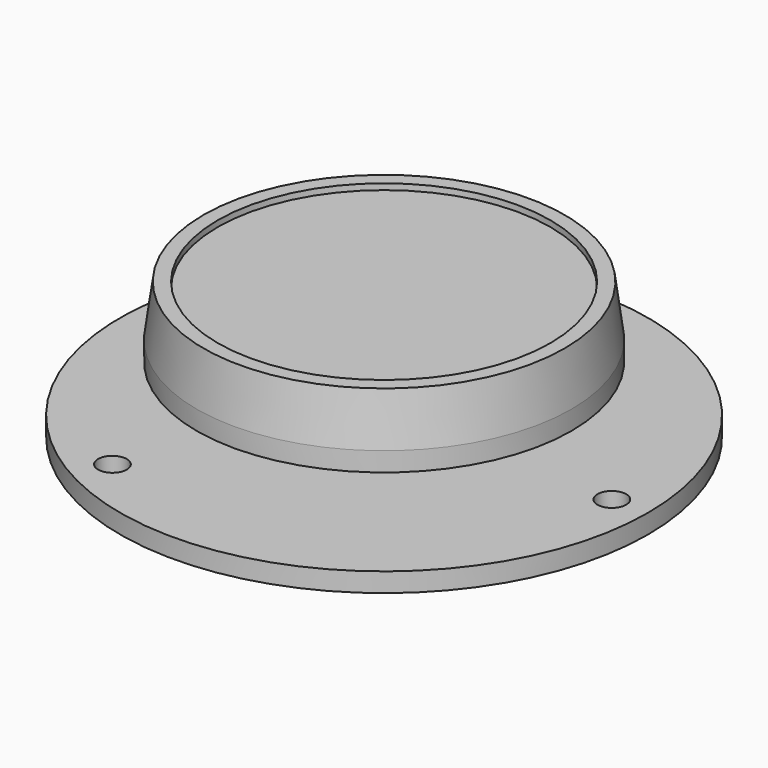
from build123d import *

# Parameters (mm, degrees)
F0_R            = 87.5
F0_R_2          = 10
F0_R_3          = 4.7625
F1_DEPTH        = 6.35
F2_DEPTH        = 6.35
F2_COPIES_COUNT = 3


# Not quite as in the source:
# - a length typed as a fraction of an inch, garbled in the dataset ("3 / 203.2 mm" for 3/8 in), is restored
# - a pattern or mirror of a feature is missing from the dataset's text; its kind, count and spacing are read off the source's solid
# - a feature names something its author has since deleted; it is built from what else it names


with BuildPart() as f1:
    # F0 (on Top) → F1 (new body)
    with BuildSketch(Plane.XY):
        Circle(F0_R)
        Circle(F0_R_2, mode=Mode.SUBTRACT)
        with Locations((75.5, 0)):
            Circle(F0_R_3, mode=Mode.SUBTRACT)
        with Locations((75.5, 0)):
            Circle(F0_R_3)
    extrude(amount=-F1_DEPTH)

    # F0 (on Top) → F2 (cut, through all)
    with BuildSketch(Plane.XY):
        with Locations((75.5, 0)):
            Circle(F0_R_3)
    f2 = extrude(amount=-F2_DEPTH, mode=Mode.SUBTRACT)

    # F2_copies: F2 ×3 about axis
    f2_copies_axis = Axis((0, 0, 0), (0, 0, 1))
    for i in range(1, F2_COPIES_COUNT):
        add(f2.rotate(f2_copies_axis, i * 360 / F2_COPIES_COUNT), mode=Mode.SUBTRACT)


with BuildPart() as f4:
    # F3 (on Front) → F4 (revolve)
    with BuildSketch(Plane.XZ):
        with BuildLine():
            ThreePointArc((0, 20.5287930104), (-12.7, 7.8287930104), (0, -4.8712069896))
            Line((0, -4.8712069896), (0, 20.5287930104))
        make_face()
    revolve(axis=Axis((0, 0, 7.8287930104), (0, 0, -1)))


with BuildPart() as f5:
    # F3 (on Front) → F5 (revolve)
    with BuildSketch(Plane.XZ):
        Polygon((0, 22.0075860208), (10, 22.0075860208), (57.15, 22.0075860208), (57.15, 37.0075860208), (55.15, 37.0075860208), (0, 37.0075860208), align=None)
    revolve(axis=Axis((0, 0, 29.5075860208), (0, 0, -1)))


with BuildPart() as f6:
    # F3 (on Front) → F6 (revolve)
    with BuildSketch(Plane.XZ):
        Polygon((10, 22.0075860208), (10, 15.6575860208), (62.15, 15.6575860208), (62.15, 22.0075860208), (59.15, 22.0075860208), (57.15, 22.0075860208), align=None)
    revolve(axis=Axis((0, 0, 7.8287930104), (0, 0, -1)))


with BuildPart() as f7:
    # F3 (on Front) → F7 (revolve)
    with BuildSketch(Plane.XZ):
        Polygon((59.15, 22.0075860208), (62.15, 22.0075860208), (59.8833333333, 39.0075860208), (55.15, 39.0075860208), (55.15, 37.0075860208), (57.15, 37.0075860208), align=None)
    revolve(axis=Axis((0, 0, 29.5075860208), (0, 0, -1)))


solid = Compound([f1.part, f4.part, f5.part, f6.part, f7.part])
